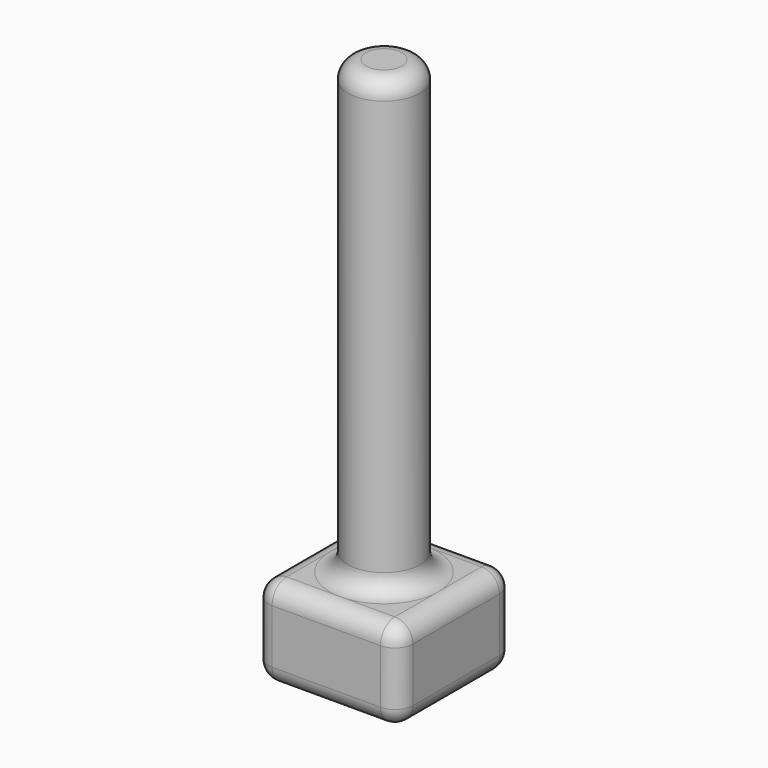
from build123d import *

# Parameters (mm, degrees)
F0_W     = 40
F0_H     = 40
F0_R     = 10
F1_DEPTH = 25
F2_DEPTH = 150
F3_R     = 4.99999


# Not quite as in the source:
# - a fillet or chamfer is up to 0.001 mm smaller than in the source, because OpenCascade refuses the exact size


with BuildPart() as f1:
    # F0 (on Top) → F1 (new body)
    with BuildSketch(Plane.XY):
        Rectangle(F0_W, F0_H)
        Circle(F0_R, mode=Mode.SUBTRACT)
    extrude(amount=F1_DEPTH)

    # F0 (on Top) → F2 (join)
    with BuildSketch(Plane.XY):
        Circle(F0_R)
    extrude(amount=F2_DEPTH)

    # F3 (radius 5 in the source; OpenCascade refuses exactly that, so slightly less here)
    f3_edges = [f1.edges().sort_by_distance(p)[0] for p in [
        (20, 0, 0),
        (0, 20, 0),
        (-20, 0, 0),
        (0, -20, 0),
        (-20, 20, 12.5),
        (-20, -20, 12.5),
        (-20, 0, 25),
        (20, -20, 12.5),
        (0, -20, 25),
        (-10, 0, 25),
        (10, 0, 87.5),
        (-10, 0, 150),
        (20, 20, 12.5),
        (20, 0, 25),
        (0, 20, 25),
    ]]
    fillet(f3_edges, radius=F3_R)


solid = f1.part
